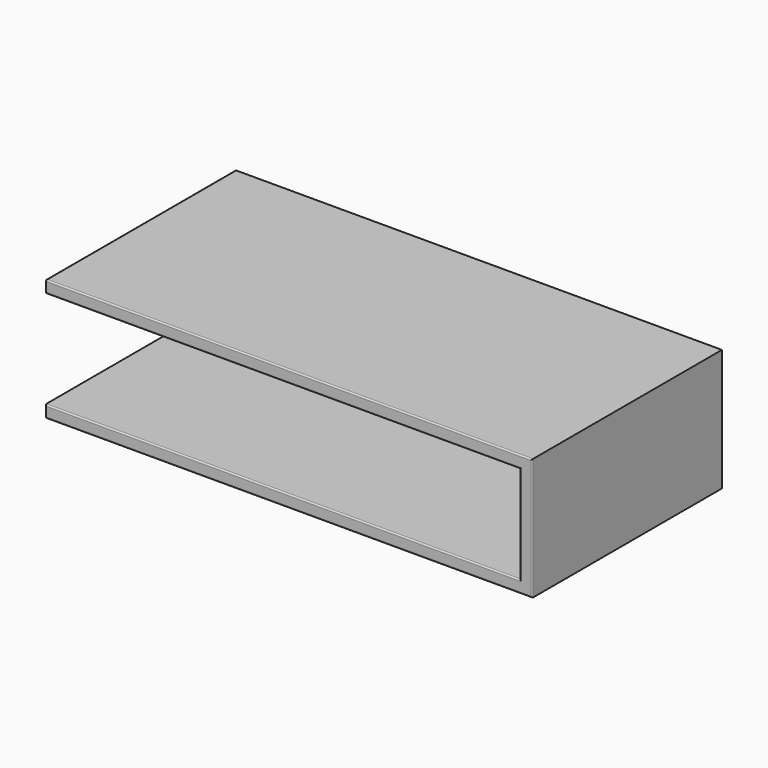
from build123d import *

# Parameters (mm, degrees)
F0_W     = 35.3801548481
F0_H     = 39.4315421581
F1_DEPTH = 350
F2_DEPTH = 718
F3_DEPTH = 180
F4_T     = -18
F5_R     = 2
F6_R     = 2


with BuildPart() as f1:
    # F0 (on Front) → F1 (new body)
    with BuildSketch(Plane.XZ):
        with Locations((17.690077424, 19.7157710791)):
            Rectangle(F0_W, F0_H)
    extrude(amount=F1_DEPTH)

    # F2 (add): a face of the model
    f2_faces = [f1.faces().sort_by_distance(p)[0] for p in [
        (0, -175, 19.7157710791),
    ]]
    extrude(f2_faces, amount=-F2_DEPTH)

    # F3 (add): a face of the model
    f3_faces = [f1.faces().sort_by_distance(p)[0] for p in [
        (359, -175, 0),
    ]]
    extrude(f3_faces, amount=-F3_DEPTH)

    # F4
    f4_openings = [f1.faces().sort_by_distance(p)[0] for p in [
        (359, -350, 90),
        (0, -175, 90),
    ]]
    offset(amount=F4_T, openings=f4_openings)

    # F5
    f5_edges = [f1.edges().sort_by_distance(p)[0] for p in [
        (359, -350, 180),
        (718, -350, 90),
        (359, -350, 0),
    ]]
    fillet(f5_edges, radius=F5_R)

    # F6
    f6_edges = [f1.edges().sort_by_distance(p)[0] for p in [
        (700, -350, 90),
        (350, -350, 162),
        (350, -350, 18),
        (0, -350, 170),
        (0, -350, 10),
        (0, -174, 0),
        (0, -174, 180),
        (0, -349.414214, 0.585786),
        (0, -349.414214, 179.414214),
    ]]
    fillet(f6_edges, radius=F6_R)


solid = f1.part
